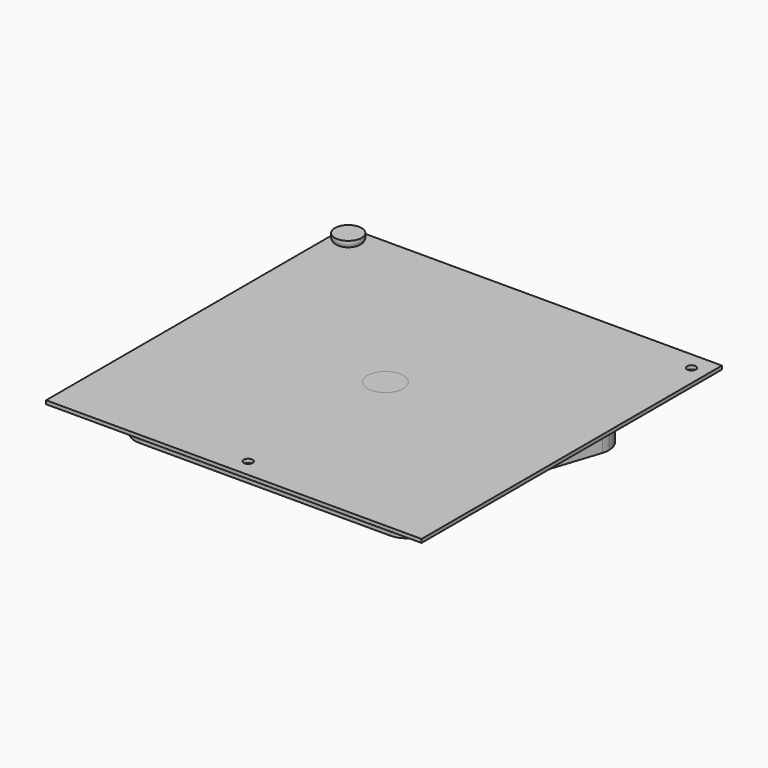
from build123d import *

# Parameters (mm, degrees)
F0_R     = 6.35
F0_R_2   = 12.7
F1_DEPTH = 12.7
F2_DEPTH = 38.1
F3_R     = 6.35
F4_DEPTH = 6.35
F5_W     = 266.7
F5_H     = 266.7
F5_R     = 9.525
F5_R_2   = 12.7
F5_R_3   = 3.175
F6_DEPTH = 2.54
F7_DEPTH = 5.08
F8_R     = 2.54


# Not quite as in the source:
# - a feature names something its author has since deleted; it is built from what else it names


with BuildPart() as f1:
    # F0 (on Top) → F1 (new body)
    with BuildSketch(Plane.XY):
        with BuildLine():
            ThreePointArc((-13.9723231754, -32.7700086168), (-19.638525588, 29.7225098602), (35.6244197099, 0))
            ThreePointArc((35.6244197099, 0), (34.7799787187, -7.7105356488), (32.2866889917, -15.0555303333))
            Line((32.2866889917, -15.0555303333), (48.5874802437, 19.9016293163))
            ThreePointArc((48.5874802437, 19.9016293163), (43.9440068681, 47.8442882261), (69.215, 35.0485491671))
            ThreePointArc((69.215, 35.0485491671), (69.018978903, 32.5615337753), (68.435756465, 30.1359366494))
            Line((68.435756465, 30.1359366494), (86.215756465, 84.7713366494))
            ThreePointArc((86.215756465, 84.7713366494), (59.5747274901, 78.7879724935), (67.0884102259, 105.0384895019))
            Line((67.0884102259, 105.0384895019), (-129.2979077289, 53.4739975689))
            ThreePointArc((-129.2979077289, 53.4739975689), (-112.8251309039, 50.1327236927), (-105.41, 35.0485491671))
            ThreePointArc((-105.41, 35.0485491671), (-113.9583857843, 19.1545692104), (-131.931637676, 17.5249328041))
            Line((-131.931637676, 17.5249328041), (-13.9723231754, -32.7700086168))
        make_face()
        with BuildLine():
            ThreePointArc((-129.2979077289, 53.4739975689), (-143.4590800142, 36.4404753919), (-131.931637676, 17.5249328041))
            ThreePointArc((-131.931637676, 17.5249328041), (-113.9583857843, 19.1545692104), (-105.41, 35.0485491671))
            ThreePointArc((-105.41, 35.0485491671), (-112.8251309039, 50.1327236927), (-129.2979077289, 53.4739975689))
        make_face()
        with Locations((-124.46, 35.0485491671)):
            Circle(F0_R, mode=Mode.SUBTRACT)
        with BuildLine():
            ThreePointArc((32.2866889917, -15.0555303333), (34.7799787187, -7.7105356488), (35.6244197099, 0))
            ThreePointArc((35.6244197099, 0), (-19.638525588, 29.7225098602), (-13.9723231754, -32.7700086168))
            ThreePointArc((-13.9723231754, -32.7700086168), (12.7398855579, -33.2685225947), (32.2866889917, -15.0555303333))
        make_face()
        Circle(F0_R_2, mode=Mode.SUBTRACT)
        with BuildLine():
            ThreePointArc((69.215, 35.0485491671), (43.9440068681, 47.8442882261), (48.5874802437, 19.9016293163))
            ThreePointArc((48.5874802437, 19.9016293163), (60.6153623999, 20.9388104399), (68.435756465, 30.1359366494))
            ThreePointArc((68.435756465, 30.1359366494), (69.018978903, 32.5615337753), (69.215, 35.0485491671))
        make_face()
        with Locations((53.34, 35.0485491671)):
            Circle(F0_R, mode=Mode.SUBTRACT)
        Circle(F0_R_2)
        with BuildLine():
            ThreePointArc((86.995, 89.6839491671), (80.8157242467, 102.2540946051), (67.0884102259, 105.0384895019))
            ThreePointArc((67.0884102259, 105.0384895019), (59.5747274901, 78.7879724935), (86.215756465, 84.7713366494))
            ThreePointArc((86.215756465, 84.7713366494), (86.798978903, 87.1969337753), (86.995, 89.6839491671))
        make_face()
        with Locations((71.12, 89.6839491671)):
            Circle(F0_R, mode=Mode.SUBTRACT)
    extrude(amount=-F1_DEPTH)

    # F0 (on Top) → F2 (join)
    with BuildSketch(Plane.XY):
        Circle(F0_R_2)
    extrude(amount=F2_DEPTH)


with BuildPart() as f4:
    # F3 (on Top) → F4 (new body)
    with BuildSketch(Plane.XY):
        with BuildLine():
            ThreePointArc((-106.4335181124, -85.2605211139), (-95.2081979611, -80.6108412652), (-90.5585181124, -69.3855211139))
            ThreePointArc((-90.5585181124, -69.3855211139), (-95.2081979611, -58.1602009625), (-106.4335181124, -53.5105211139))
            ThreePointArc((-106.4335181124, -53.5105211139), (-122.3085181124, -69.3855211139), (-106.4335181124, -85.2605211139))
        make_face()
        with Locations((-106.4335181124, -69.3855211139)):
            Circle(F3_R, mode=Mode.SUBTRACT)
        with BuildLine():
            ThreePointArc((-106.4335181124, -53.5105211139), (-95.2081979611, -58.1602009625), (-90.5585181124, -69.3855211139))
            ThreePointArc((-90.5585181124, -69.3855211139), (-95.2081979611, -80.6108412652), (-106.4335181124, -85.2605211139))
            Line((-106.4335181124, -85.2605211139), (71.3664818876, -85.2605211139))
            ThreePointArc((71.3664818876, -85.2605211139), (55.4914818876, -69.3855211139), (71.3664818876, -53.5105211139))
            Line((71.3664818876, -53.5105211139), (-106.4335181124, -53.5105211139))
        make_face()
        with BuildLine():
            ThreePointArc((87.2414818876, -69.3855211139), (82.5918020389, -58.1602009625), (71.3664818876, -53.5105211139))
            ThreePointArc((71.3664818876, -53.5105211139), (55.4914818876, -69.3855211139), (71.3664818876, -85.2605211139))
            ThreePointArc((71.3664818876, -85.2605211139), (82.5918020389, -80.6108412652), (87.2414818876, -69.3855211139))
        make_face()
        with Locations((71.3664818876, -69.3855211139)):
            Circle(F3_R, mode=Mode.SUBTRACT)
    extrude(amount=F4_DEPTH)


with BuildPart() as f6:
    # F5 (on face) → F6 (new body)
    with BuildSketch(Plane.XY.offset(38.1)):
        with Locations((0, -1.27)):
            Rectangle(F5_W, F5_H)
        with Locations((0, -121.92)):
            Circle(F5_R, mode=Mode.SUBTRACT)
        with Locations((-121.92, 119.38)):
            Circle(F5_R, mode=Mode.SUBTRACT)
        Circle(F5_R_2, mode=Mode.SUBTRACT)
        with Locations((121.92, 119.38)):
            Circle(F5_R, mode=Mode.SUBTRACT)
        with Locations((-121.92, 119.38)):
            Circle(F5_R)
        with Locations((-121.92, 119.38)):
            Circle(F5_R_3, mode=Mode.SUBTRACT)
        with Locations((121.92, 119.38)):
            Circle(F5_R)
        with Locations((121.92, 119.38)):
            Circle(F5_R_3, mode=Mode.SUBTRACT)
        with Locations((0, -121.92)):
            Circle(F5_R)
        with Locations((0, -121.92)):
            Circle(F5_R_3, mode=Mode.SUBTRACT)
    extrude(amount=-F6_DEPTH)


with BuildPart() as f7:
    # F5 (on face) → F7 (new body)
    with BuildSketch(Plane.XY.offset(38.1)):
        with Locations((-121.92, 119.38)):
            Circle(F5_R)
        with Locations((-121.92, 119.38)):
            Circle(F5_R_3, mode=Mode.SUBTRACT)
        with Locations((-121.92, 119.38)):
            Circle(F5_R_3)
    extrude(amount=F7_DEPTH)

    # F8
    f8_edges = [f7.edges().sort_by_distance(p)[0] for p in [
        (-131.445, 119.38, 38.1),
    ]]
    fillet(f8_edges, radius=F8_R)


solid = Compound([f1.part, f4.part, f6.part, f7.part])
